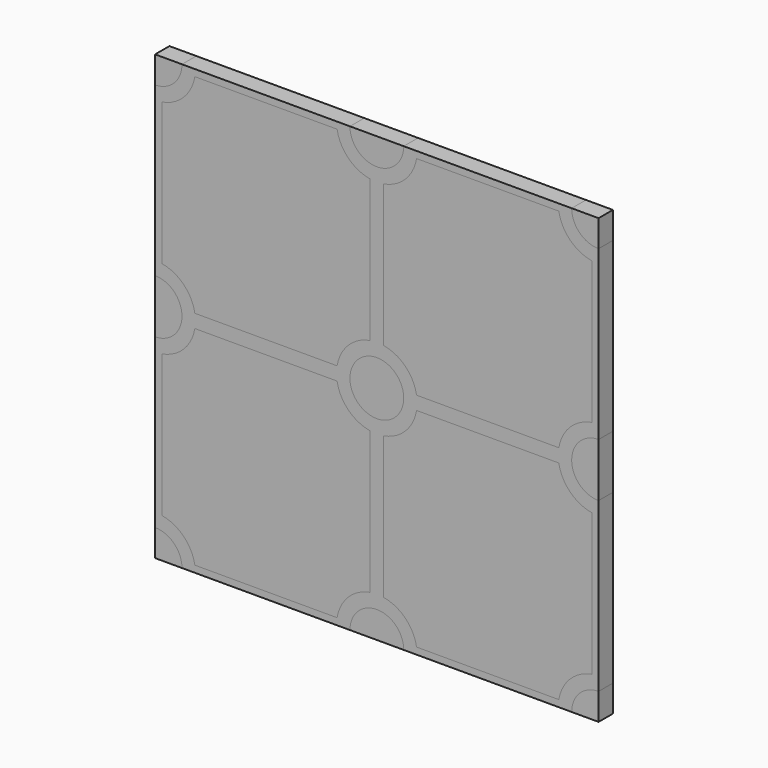
from build123d import *

# Parameters (mm, degrees)
F2_DEPTH = 6.35
F3_DEPTH = 6.35
F1_W     = 4.7625
F1_H     = 4.7625
F4_DEPTH = 6.35


with BuildPart() as f2:
    # F1 (on face) → F2 (new body)
    with BuildSketch(Plane.XZ):
        with BuildLine():
            Line((-64.4935850165, 2.38125), (-14.0876649835, 2.38125))
            ThreePointArc((-14.0876649835, 2.38125), (-10.1027881362, 10.1027881362), (-2.38125, 14.0876649835))
            Line((-2.38125, 14.0876649835), (-2.38125, 64.4935850165))
            ThreePointArc((-2.38125, 64.4935850165), (-10.1027881362, 68.4784618638), (-14.0876649835, 76.2))
            Line((-14.0876649835, 76.2), (-64.4935850165, 76.2))
            ThreePointArc((-64.4935850165, 76.2), (-68.4784618638, 68.4784618638), (-76.2, 64.4935850165))
            Line((-76.2, 64.4935850165), (-76.2, 14.0876649835))
            ThreePointArc((-76.2, 14.0876649835), (-68.4784618638, 10.1027881362), (-64.4935850165, 2.38125))
        make_face()
    extrude(amount=F2_DEPTH)


with BuildPart() as f2b:
    # F1 (on face) → F2, piece 2 (new body)
    with BuildSketch(Plane.XZ):
        with BuildLine():
            Line((14.0876649835, 2.38125), (64.4935850165, 2.38125))
            ThreePointArc((64.4935850165, 2.38125), (68.4784618638, 10.1027881362), (76.2, 14.0876649835))
            Line((76.2, 14.0876649835), (76.2, 64.4935850165))
            ThreePointArc((76.2, 64.4935850165), (68.4784618638, 68.4784618638), (64.4935850165, 76.2))
            Line((64.4935850165, 76.2), (14.0876649835, 76.2))
            ThreePointArc((14.0876649835, 76.2), (10.1027881362, 68.4784618638), (2.38125, 64.4935850165))
            Line((2.38125, 64.4935850165), (2.38125, 14.0876649835))
            ThreePointArc((2.38125, 14.0876649835), (10.1027881362, 10.1027881362), (14.0876649835, 2.38125))
        make_face()
    extrude(amount=F2_DEPTH)


with BuildPart() as f2c:
    # F1 (on face) → F2, piece 3 (new body)
    with BuildSketch(Plane.XZ):
        with BuildLine():
            Line((-64.4935850165, -76.2), (-14.0876649835, -76.2))
            ThreePointArc((-14.0876649835, -76.2), (-10.1027881362, -68.4784618638), (-2.38125, -64.4935850165))
            Line((-2.38125, -64.4935850165), (-2.38125, -14.0876649835))
            ThreePointArc((-2.38125, -14.0876649835), (-10.1027881362, -10.1027881362), (-14.0876649835, -2.38125))
            Line((-14.0876649835, -2.38125), (-64.4935850165, -2.38125))
            ThreePointArc((-64.4935850165, -2.38125), (-68.4784618638, -10.1027881362), (-76.2, -14.0876649835))
            Line((-76.2, -14.0876649835), (-76.2, -64.4935850165))
            ThreePointArc((-76.2, -64.4935850165), (-68.4784618638, -68.4784618638), (-64.4935850165, -76.2))
        make_face()
    extrude(amount=F2_DEPTH)


with BuildPart() as f2d:
    # F1 (on face) → F2, piece 4 (new body)
    with BuildSketch(Plane.XZ):
        with BuildLine():
            ThreePointArc((2.38125, -64.4935850165), (10.1027881362, -68.4784618638), (14.0876649835, -76.2))
            Line((14.0876649835, -76.2), (64.4935850165, -76.2))
            ThreePointArc((64.4935850165, -76.2), (68.4784618638, -68.4784618638), (76.2, -64.4935850165))
            Line((76.2, -64.4935850165), (76.2, -14.0876649835))
            ThreePointArc((76.2, -14.0876649835), (68.4784618638, -10.1027881362), (64.4935850165, -2.38125))
            Line((64.4935850165, -2.38125), (14.0876649835, -2.38125))
            ThreePointArc((14.0876649835, -2.38125), (10.1027881362, -10.1027881362), (2.38125, -14.0876649835))
            Line((2.38125, -14.0876649835), (2.38125, -64.4935850165))
        make_face()
    extrude(amount=F2_DEPTH)


with BuildPart() as f3:
    # F1 (on face) → F3 (new body)
    with BuildSketch(Plane.XZ):
        with BuildLine():
            Line((-76.2, 76.2), (-76.2, 69.3587084068))
            ThreePointArc((-76.2, 69.3587084068), (-71.8460579092, 71.8460579092), (-69.3587084068, 76.2))
            Line((-69.3587084068, 76.2), (-76.2, 76.2))
        make_face()
        with BuildLine():
            Line((-78.58125, 78.58125), (-78.58125, 69.05625))
            ThreePointArc((-78.58125, 69.05625), (-77.3810591141, 69.1321671431), (-76.2, 69.3587084068))
            Line((-76.2, 69.3587084068), (-76.2, 76.2))
            Line((-76.2, 76.2), (-69.3587084068, 76.2))
            ThreePointArc((-69.3587084068, 76.2), (-69.1321671431, 77.3810591141), (-69.05625, 78.58125))
            Line((-69.05625, 78.58125), (-78.58125, 78.58125))
        make_face()
    extrude(amount=F3_DEPTH)


with BuildPart() as f3b:
    # F1 (on face) → F3, piece 2 (new body)
    with BuildSketch(Plane.XZ):
        with BuildLine():
            Line((9.525, 78.58125), (-9.525, 78.58125))
            ThreePointArc((-9.525, 78.58125), (-9.4490828569, 77.3810591141), (-9.2225415932, 76.2))
            Line((-9.2225415932, 76.2), (-2.38125, 76.2))
            Line((-2.38125, 76.2), (2.38125, 76.2))
            Line((2.38125, 76.2), (9.2225415932, 76.2))
            ThreePointArc((9.2225415932, 76.2), (9.4490828569, 77.3810591141), (9.525, 78.58125))
        make_face()
        with BuildLine():
            ThreePointArc((-9.2225415932, 76.2), (-6.7351920908, 71.8460579092), (-2.38125, 69.3587084068))
            Line((-2.38125, 69.3587084068), (-2.38125, 76.2))
            Line((-2.38125, 76.2), (-9.2225415932, 76.2))
        make_face()
        with BuildLine():
            Line((-2.38125, 76.2), (-2.38125, 69.3587084068))
            ThreePointArc((-2.38125, 69.3587084068), (0, 69.05625), (2.38125, 69.3587084068))
            Line((2.38125, 69.3587084068), (2.38125, 76.2))
            Line((2.38125, 76.2), (-2.38125, 76.2))
        make_face()
        with BuildLine():
            Line((2.38125, 76.2), (2.38125, 69.3587084068))
            ThreePointArc((2.38125, 69.3587084068), (6.7351920908, 71.8460579092), (9.2225415932, 76.2))
            Line((9.2225415932, 76.2), (2.38125, 76.2))
        make_face()
    extrude(amount=F3_DEPTH)


with BuildPart() as f3c:
    # F1 (on face) → F3, piece 3 (new body)
    with BuildSketch(Plane.XZ):
        with BuildLine():
            ThreePointArc((69.3587084068, 76.2), (71.8460579092, 71.8460579092), (76.2, 69.3587084068))
            Line((76.2, 69.3587084068), (76.2, 76.2))
            Line((76.2, 76.2), (69.3587084068, 76.2))
        make_face()
        with BuildLine():
            ThreePointArc((76.2, 69.3587084068), (77.3810591141, 69.1321671431), (78.58125, 69.05625))
            Line((78.58125, 69.05625), (78.58125, 78.58125))
            Line((78.58125, 78.58125), (69.05625, 78.58125))
            ThreePointArc((69.05625, 78.58125), (69.1321671431, 77.3810591141), (69.3587084068, 76.2))
            Line((69.3587084068, 76.2), (76.2, 76.2))
            Line((76.2, 76.2), (76.2, 69.3587084068))
        make_face()
    extrude(amount=F3_DEPTH)


with BuildPart() as f3d:
    # F1 (on face) → F3, piece 4 (new body)
    with BuildSketch(Plane.XZ):
        with BuildLine():
            Line((69.3587084068, 2.38125), (76.2, 2.38125))
            Line((76.2, 2.38125), (76.2, 9.2225415932))
            ThreePointArc((76.2, 9.2225415932), (71.8460579092, 6.7351920908), (69.3587084068, 2.38125))
        make_face()
        with BuildLine():
            Line((76.2, -2.38125), (76.2, -9.2225415932))
            ThreePointArc((76.2, -9.2225415932), (77.3810591141, -9.4490828569), (78.58125, -9.525))
            Line((78.58125, -9.525), (78.58125, 9.525))
            ThreePointArc((78.58125, 9.525), (77.3810591141, 9.4490828569), (76.2, 9.2225415932))
            Line((76.2, 9.2225415932), (76.2, 2.38125))
            Line((76.2, 2.38125), (76.2, -2.38125))
        make_face()
        with BuildLine():
            Line((69.3587084068, -2.38125), (76.2, -2.38125))
            Line((76.2, -2.38125), (76.2, 2.38125))
            Line((76.2, 2.38125), (69.3587084068, 2.38125))
            ThreePointArc((69.3587084068, 2.38125), (69.05625, 0), (69.3587084068, -2.38125))
        make_face()
        with BuildLine():
            ThreePointArc((69.3587084068, -2.38125), (71.8460579092, -6.7351920908), (76.2, -9.2225415932))
            Line((76.2, -9.2225415932), (76.2, -2.38125))
            Line((76.2, -2.38125), (69.3587084068, -2.38125))
        make_face()
    extrude(amount=F3_DEPTH)


with BuildPart() as f3e:
    # F1 (on face) → F3, piece 5 (new body)
    with BuildSketch(Plane.XZ):
        with BuildLine():
            ThreePointArc((76.2, -69.3587084068), (71.8460579092, -71.8460579092), (69.3587084068, -76.2))
            Line((69.3587084068, -76.2), (76.2, -76.2))
            Line((76.2, -76.2), (76.2, -69.3587084068))
        make_face()
        with BuildLine():
            ThreePointArc((69.3587084068, -76.2), (69.1321671431, -77.3810591141), (69.05625, -78.58125))
            Line((69.05625, -78.58125), (78.58125, -78.58125))
            Line((78.58125, -78.58125), (78.58125, -69.05625))
            ThreePointArc((78.58125, -69.05625), (77.3810591141, -69.1321671431), (76.2, -69.3587084068))
            Line((76.2, -69.3587084068), (76.2, -76.2))
            Line((76.2, -76.2), (69.3587084068, -76.2))
        make_face()
    extrude(amount=F3_DEPTH)


with BuildPart() as f3f:
    # F1 (on face) → F3, piece 6 (new body)
    with BuildSketch(Plane.XZ):
        with BuildLine():
            Line((2.38125, -76.2), (9.2225415932, -76.2))
            ThreePointArc((9.2225415932, -76.2), (6.7351920908, -71.8460579092), (2.38125, -69.3587084068))
            Line((2.38125, -69.3587084068), (2.38125, -76.2))
        make_face()
        with BuildLine():
            ThreePointArc((-2.38125, -69.3587084068), (-6.7351920908, -71.8460579092), (-9.2225415932, -76.2))
            Line((-9.2225415932, -76.2), (-2.38125, -76.2))
            Line((-2.38125, -76.2), (-2.38125, -69.3587084068))
        make_face()
        with BuildLine():
            Line((-9.525, -78.58125), (9.525, -78.58125))
            ThreePointArc((9.525, -78.58125), (9.4490828569, -77.3810591141), (9.2225415932, -76.2))
            Line((9.2225415932, -76.2), (2.38125, -76.2))
            Line((2.38125, -76.2), (-2.38125, -76.2))
            Line((-2.38125, -76.2), (-9.2225415932, -76.2))
            ThreePointArc((-9.2225415932, -76.2), (-9.4490828569, -77.3810591141), (-9.525, -78.58125))
        make_face()
        with BuildLine():
            Line((-2.38125, -76.2), (2.38125, -76.2))
            Line((2.38125, -76.2), (2.38125, -69.3587084068))
            ThreePointArc((2.38125, -69.3587084068), (0, -69.05625), (-2.38125, -69.3587084068))
            Line((-2.38125, -69.3587084068), (-2.38125, -76.2))
        make_face()
    extrude(amount=F3_DEPTH)


with BuildPart() as f3g:
    # F1 (on face) → F3, piece 7 (new body)
    with BuildSketch(Plane.XZ):
        with BuildLine():
            Line((2.38125, -2.38125), (2.38125, -9.2225415932))
            ThreePointArc((2.38125, -9.2225415932), (6.7351920908, -6.7351920908), (9.2225415932, -2.38125))
            Line((9.2225415932, -2.38125), (2.38125, -2.38125))
        make_face()
        with BuildLine():
            ThreePointArc((-2.38125, -9.2225415932), (0, -9.525), (2.38125, -9.2225415932))
            Line((2.38125, -9.2225415932), (2.38125, -2.38125))
            Line((2.38125, -2.38125), (-2.38125, -2.38125))
            Line((-2.38125, -2.38125), (-2.38125, -9.2225415932))
        make_face()
        with BuildLine():
            ThreePointArc((-9.2225415932, -2.38125), (-6.7351920908, -6.7351920908), (-2.38125, -9.2225415932))
            Line((-2.38125, -9.2225415932), (-2.38125, -2.38125))
            Line((-2.38125, -2.38125), (-9.2225415932, -2.38125))
        make_face()
        with BuildLine():
            ThreePointArc((-9.2225415932, 2.38125), (-9.525, 0), (-9.2225415932, -2.38125))
            Line((-9.2225415932, -2.38125), (-2.38125, -2.38125))
            Line((-2.38125, -2.38125), (-2.38125, 2.38125))
            Line((-2.38125, 2.38125), (-9.2225415932, 2.38125))
        make_face()
        with BuildLine():
            ThreePointArc((-2.38125, 9.2225415932), (-6.7351920908, 6.7351920908), (-9.2225415932, 2.38125))
            Line((-9.2225415932, 2.38125), (-2.38125, 2.38125))
            Line((-2.38125, 2.38125), (-2.38125, 9.2225415932))
        make_face()
        with BuildLine():
            Line((-2.38125, 2.38125), (2.38125, 2.38125))
            Line((2.38125, 2.38125), (2.38125, 9.2225415932))
            ThreePointArc((2.38125, 9.2225415932), (0, 9.525), (-2.38125, 9.2225415932))
            Line((-2.38125, 9.2225415932), (-2.38125, 2.38125))
        make_face()
        with BuildLine():
            Line((2.38125, 9.2225415932), (2.38125, 2.38125))
            Line((2.38125, 2.38125), (9.2225415932, 2.38125))
            ThreePointArc((9.2225415932, 2.38125), (6.7351920908, 6.7351920908), (2.38125, 9.2225415932))
        make_face()
        with BuildLine():
            Line((2.38125, -2.38125), (9.2225415932, -2.38125))
            ThreePointArc((9.2225415932, -2.38125), (9.4490828569, -1.2001908859), (9.525, 0))
            ThreePointArc((9.525, 0), (9.4490828569, 1.2001908859), (9.2225415932, 2.38125))
            Line((9.2225415932, 2.38125), (2.38125, 2.38125))
            Line((2.38125, 2.38125), (2.38125, -2.38125))
        make_face()
        Rectangle(F1_W, F1_H)
    extrude(amount=F3_DEPTH)


with BuildPart() as f3h:
    # F1 (on face) → F3, piece 8 (new body)
    with BuildSketch(Plane.XZ):
        with BuildLine():
            Line((-76.2, -76.2), (-69.3587084068, -76.2))
            ThreePointArc((-69.3587084068, -76.2), (-71.8460579092, -71.8460579092), (-76.2, -69.3587084068))
            Line((-76.2, -69.3587084068), (-76.2, -76.2))
        make_face()
        with BuildLine():
            Line((-78.58125, -78.58125), (-69.05625, -78.58125))
            ThreePointArc((-69.05625, -78.58125), (-69.1321671431, -77.3810591141), (-69.3587084068, -76.2))
            Line((-69.3587084068, -76.2), (-76.2, -76.2))
            Line((-76.2, -76.2), (-76.2, -69.3587084068))
            ThreePointArc((-76.2, -69.3587084068), (-77.3810591141, -69.1321671431), (-78.58125, -69.05625))
            Line((-78.58125, -69.05625), (-78.58125, -78.58125))
        make_face()
    extrude(amount=F3_DEPTH)


with BuildPart() as f3i:
    # F1 (on face) → F3, piece 9 (new body)
    with BuildSketch(Plane.XZ):
        with BuildLine():
            Line((-76.2, -2.38125), (-76.2, -9.2225415932))
            ThreePointArc((-76.2, -9.2225415932), (-71.8460579092, -6.7351920908), (-69.3587084068, -2.38125))
            Line((-69.3587084068, -2.38125), (-76.2, -2.38125))
        make_face()
        with BuildLine():
            Line((-78.58125, 9.525), (-78.58125, -9.525))
            ThreePointArc((-78.58125, -9.525), (-77.3810591141, -9.4490828569), (-76.2, -9.2225415932))
            Line((-76.2, -9.2225415932), (-76.2, -2.38125))
            Line((-76.2, -2.38125), (-76.2, 2.38125))
            Line((-76.2, 2.38125), (-76.2, 9.2225415932))
            ThreePointArc((-76.2, 9.2225415932), (-77.3810591141, 9.4490828569), (-78.58125, 9.525))
        make_face()
        with BuildLine():
            Line((-76.2, -2.38125), (-69.3587084068, -2.38125))
            ThreePointArc((-69.3587084068, -2.38125), (-69.1321671431, -1.2001908859), (-69.05625, 0))
            ThreePointArc((-69.05625, 0), (-69.1321671431, 1.2001908859), (-69.3587084068, 2.38125))
            Line((-69.3587084068, 2.38125), (-76.2, 2.38125))
            Line((-76.2, 2.38125), (-76.2, -2.38125))
        make_face()
        with BuildLine():
            ThreePointArc((-69.3587084068, 2.38125), (-71.8460579092, 6.7351920908), (-76.2, 9.2225415932))
            Line((-76.2, 9.2225415932), (-76.2, 2.38125))
            Line((-76.2, 2.38125), (-69.3587084068, 2.38125))
        make_face()
    extrude(amount=F3_DEPTH)


with BuildPart() as f4:
    # F1 (on face) → F4 (new body)
    with BuildSketch(Plane.XZ):
        with BuildLine():
            ThreePointArc((-64.4935850165, 76.2), (-64.3437964057, 77.3864398063), (-64.29375, 78.58125))
            Line((-64.29375, 78.58125), (-69.05625, 78.58125))
            ThreePointArc((-69.05625, 78.58125), (-69.1321671431, 77.3810591141), (-69.3587084068, 76.2))
            Line((-69.3587084068, 76.2), (-64.4935850165, 76.2))
        make_face()
        with BuildLine():
            Line((-76.2, 69.3587084068), (-76.2, 64.4935850165))
            ThreePointArc((-76.2, 64.4935850165), (-68.4784618638, 68.4784618638), (-64.4935850165, 76.2))
            Line((-64.4935850165, 76.2), (-69.3587084068, 76.2))
            ThreePointArc((-69.3587084068, 76.2), (-71.8460579092, 71.8460579092), (-76.2, 69.3587084068))
        make_face()
        with BuildLine():
            Line((-78.58125, 69.05625), (-78.58125, 64.29375))
            ThreePointArc((-78.58125, 64.29375), (-77.3864398063, 64.3437964057), (-76.2, 64.4935850165))
            Line((-76.2, 64.4935850165), (-76.2, 69.3587084068))
            ThreePointArc((-76.2, 69.3587084068), (-77.3810591141, 69.1321671431), (-78.58125, 69.05625))
        make_face()
        with BuildLine():
            Line((-78.58125, 64.29375), (-78.58125, 14.2875))
            ThreePointArc((-78.58125, 14.2875), (-77.3864398063, 14.2374535943), (-76.2, 14.0876649835))
            Line((-76.2, 14.0876649835), (-76.2, 64.4935850165))
            ThreePointArc((-76.2, 64.4935850165), (-77.3864398063, 64.3437964057), (-78.58125, 64.29375))
        make_face()
        with BuildLine():
            ThreePointArc((-76.2, 14.0876649835), (-77.3864398063, 14.2374535943), (-78.58125, 14.2875))
            Line((-78.58125, 14.2875), (-78.58125, 9.525))
            ThreePointArc((-78.58125, 9.525), (-77.3810591141, 9.4490828569), (-76.2, 9.2225415932))
            Line((-76.2, 9.2225415932), (-76.2, 14.0876649835))
        make_face()
        with BuildLine():
            ThreePointArc((-64.4935850165, 2.38125), (-68.4784618638, 10.1027881362), (-76.2, 14.0876649835))
            Line((-76.2, 14.0876649835), (-76.2, 9.2225415932))
            ThreePointArc((-76.2, 9.2225415932), (-71.8460579092, 6.7351920908), (-69.3587084068, 2.38125))
            Line((-69.3587084068, 2.38125), (-64.4935850165, 2.38125))
        make_face()
        with BuildLine():
            Line((-69.3587084068, -2.38125), (-64.4935850165, -2.38125))
            ThreePointArc((-64.4935850165, -2.38125), (-64.3437964057, -1.1948101937), (-64.29375, 0))
            ThreePointArc((-64.29375, 0), (-64.3437964057, 1.1948101937), (-64.4935850165, 2.38125))
            Line((-64.4935850165, 2.38125), (-69.3587084068, 2.38125))
            ThreePointArc((-69.3587084068, 2.38125), (-69.1321671431, 1.2001908859), (-69.05625, 0))
            ThreePointArc((-69.05625, 0), (-69.1321671431, -1.2001908859), (-69.3587084068, -2.38125))
        make_face()
        with BuildLine():
            Line((-76.2, -9.2225415932), (-76.2, -14.0876649835))
            ThreePointArc((-76.2, -14.0876649835), (-68.4784618638, -10.1027881362), (-64.4935850165, -2.38125))
            Line((-64.4935850165, -2.38125), (-69.3587084068, -2.38125))
            ThreePointArc((-69.3587084068, -2.38125), (-71.8460579092, -6.7351920908), (-76.2, -9.2225415932))
        make_face()
        with BuildLine():
            Line((-64.4935850165, -2.38125), (-14.0876649835, -2.38125))
            ThreePointArc((-14.0876649835, -2.38125), (-14.2875, 0), (-14.0876649835, 2.38125))
            Line((-14.0876649835, 2.38125), (-64.4935850165, 2.38125))
            ThreePointArc((-64.4935850165, 2.38125), (-64.3437964057, 1.1948101937), (-64.29375, 0))
            ThreePointArc((-64.29375, 0), (-64.3437964057, -1.1948101937), (-64.4935850165, -2.38125))
        make_face()
        with BuildLine():
            ThreePointArc((-2.38125, 14.0876649835), (-10.1027881362, 10.1027881362), (-14.0876649835, 2.38125))
            Line((-14.0876649835, 2.38125), (-9.2225415932, 2.38125))
            ThreePointArc((-9.2225415932, 2.38125), (-6.7351920908, 6.7351920908), (-2.38125, 9.2225415932))
            Line((-2.38125, 9.2225415932), (-2.38125, 14.0876649835))
        make_face()
        with BuildLine():
            ThreePointArc((-14.0876649835, 2.38125), (-14.2875, 0), (-14.0876649835, -2.38125))
            Line((-14.0876649835, -2.38125), (-9.2225415932, -2.38125))
            ThreePointArc((-9.2225415932, -2.38125), (-9.525, 0), (-9.2225415932, 2.38125))
            Line((-9.2225415932, 2.38125), (-14.0876649835, 2.38125))
        make_face()
        with BuildLine():
            ThreePointArc((-14.0876649835, -2.38125), (-10.1027881362, -10.1027881362), (-2.38125, -14.0876649835))
            Line((-2.38125, -14.0876649835), (-2.38125, -9.2225415932))
            ThreePointArc((-2.38125, -9.2225415932), (-6.7351920908, -6.7351920908), (-9.2225415932, -2.38125))
            Line((-9.2225415932, -2.38125), (-14.0876649835, -2.38125))
        make_face()
        with BuildLine():
            ThreePointArc((-2.38125, -14.0876649835), (0, -14.2875), (2.38125, -14.0876649835))
            Line((2.38125, -14.0876649835), (2.38125, -9.2225415932))
            ThreePointArc((2.38125, -9.2225415932), (0, -9.525), (-2.38125, -9.2225415932))
            Line((-2.38125, -9.2225415932), (-2.38125, -14.0876649835))
        make_face()
        with BuildLine():
            Line((2.38125, -9.2225415932), (2.38125, -14.0876649835))
            ThreePointArc((2.38125, -14.0876649835), (10.1027881362, -10.1027881362), (14.0876649835, -2.38125))
            Line((14.0876649835, -2.38125), (9.2225415932, -2.38125))
            ThreePointArc((9.2225415932, -2.38125), (6.7351920908, -6.7351920908), (2.38125, -9.2225415932))
        make_face()
        with BuildLine():
            Line((9.2225415932, 2.38125), (14.0876649835, 2.38125))
            ThreePointArc((14.0876649835, 2.38125), (10.1027881362, 10.1027881362), (2.38125, 14.0876649835))
            Line((2.38125, 14.0876649835), (2.38125, 9.2225415932))
            ThreePointArc((2.38125, 9.2225415932), (6.7351920908, 6.7351920908), (9.2225415932, 2.38125))
        make_face()
        with BuildLine():
            Line((9.2225415932, -2.38125), (14.0876649835, -2.38125))
            ThreePointArc((14.0876649835, -2.38125), (14.2374535943, -1.1948101937), (14.2875, 0))
            ThreePointArc((14.2875, 0), (14.2374535943, 1.1948101937), (14.0876649835, 2.38125))
            Line((14.0876649835, 2.38125), (9.2225415932, 2.38125))
            ThreePointArc((9.2225415932, 2.38125), (9.4490828569, 1.2001908859), (9.525, 0))
            ThreePointArc((9.525, 0), (9.4490828569, -1.2001908859), (9.2225415932, -2.38125))
        make_face()
        with BuildLine():
            ThreePointArc((2.38125, 14.0876649835), (0, 14.2875), (-2.38125, 14.0876649835))
            Line((-2.38125, 14.0876649835), (-2.38125, 9.2225415932))
            ThreePointArc((-2.38125, 9.2225415932), (0, 9.525), (2.38125, 9.2225415932))
            Line((2.38125, 9.2225415932), (2.38125, 14.0876649835))
        make_face()
        with BuildLine():
            Line((-2.38125, 64.4935850165), (-2.38125, 14.0876649835))
            ThreePointArc((-2.38125, 14.0876649835), (0, 14.2875), (2.38125, 14.0876649835))
            Line((2.38125, 14.0876649835), (2.38125, 64.4935850165))
            ThreePointArc((2.38125, 64.4935850165), (0, 64.29375), (-2.38125, 64.4935850165))
        make_face()
        with BuildLine():
            ThreePointArc((-14.0876649835, 76.2), (-10.1027881362, 68.4784618638), (-2.38125, 64.4935850165))
            Line((-2.38125, 64.4935850165), (-2.38125, 69.3587084068))
            ThreePointArc((-2.38125, 69.3587084068), (-6.7351920908, 71.8460579092), (-9.2225415932, 76.2))
            Line((-9.2225415932, 76.2), (-14.0876649835, 76.2))
        make_face()
        with BuildLine():
            Line((-2.38125, 69.3587084068), (-2.38125, 64.4935850165))
            ThreePointArc((-2.38125, 64.4935850165), (0, 64.29375), (2.38125, 64.4935850165))
            Line((2.38125, 64.4935850165), (2.38125, 69.3587084068))
            ThreePointArc((2.38125, 69.3587084068), (0, 69.05625), (-2.38125, 69.3587084068))
        make_face()
        with BuildLine():
            Line((2.38125, 69.3587084068), (2.38125, 64.4935850165))
            ThreePointArc((2.38125, 64.4935850165), (10.1027881362, 68.4784618638), (14.0876649835, 76.2))
            Line((14.0876649835, 76.2), (9.2225415932, 76.2))
            ThreePointArc((9.2225415932, 76.2), (6.7351920908, 71.8460579092), (2.38125, 69.3587084068))
        make_face()
        with BuildLine():
            Line((-9.525, 78.58125), (-14.2875, 78.58125))
            ThreePointArc((-14.2875, 78.58125), (-14.2374535943, 77.3864398063), (-14.0876649835, 76.2))
            Line((-14.0876649835, 76.2), (-9.2225415932, 76.2))
            ThreePointArc((-9.2225415932, 76.2), (-9.4490828569, 77.3810591141), (-9.525, 78.58125))
        make_face()
        with BuildLine():
            Line((-14.2875, 78.58125), (-64.29375, 78.58125))
            ThreePointArc((-64.29375, 78.58125), (-64.3437964057, 77.3864398063), (-64.4935850165, 76.2))
            Line((-64.4935850165, 76.2), (-14.0876649835, 76.2))
            ThreePointArc((-14.0876649835, 76.2), (-14.2374535943, 77.3864398063), (-14.2875, 78.58125))
        make_face()
        with BuildLine():
            Line((9.2225415932, 76.2), (14.0876649835, 76.2))
            ThreePointArc((14.0876649835, 76.2), (14.2374535943, 77.3864398063), (14.2875, 78.58125))
            Line((14.2875, 78.58125), (9.525, 78.58125))
            ThreePointArc((9.525, 78.58125), (9.4490828569, 77.3810591141), (9.2225415932, 76.2))
        make_face()
        with BuildLine():
            Line((14.0876649835, 76.2), (64.4935850165, 76.2))
            ThreePointArc((64.4935850165, 76.2), (64.3437964057, 77.3864398063), (64.29375, 78.58125))
            Line((64.29375, 78.58125), (14.2875, 78.58125))
            ThreePointArc((14.2875, 78.58125), (14.2374535943, 77.3864398063), (14.0876649835, 76.2))
        make_face()
        with BuildLine():
            ThreePointArc((64.29375, 78.58125), (64.3437964057, 77.3864398063), (64.4935850165, 76.2))
            Line((64.4935850165, 76.2), (69.3587084068, 76.2))
            ThreePointArc((69.3587084068, 76.2), (69.1321671431, 77.3810591141), (69.05625, 78.58125))
            Line((69.05625, 78.58125), (64.29375, 78.58125))
        make_face()
        with BuildLine():
            ThreePointArc((64.4935850165, 76.2), (68.4784618638, 68.4784618638), (76.2, 64.4935850165))
            Line((76.2, 64.4935850165), (76.2, 69.3587084068))
            ThreePointArc((76.2, 69.3587084068), (71.8460579092, 71.8460579092), (69.3587084068, 76.2))
            Line((69.3587084068, 76.2), (64.4935850165, 76.2))
        make_face()
        with BuildLine():
            ThreePointArc((76.2, 64.4935850165), (77.3864398063, 64.3437964057), (78.58125, 64.29375))
            Line((78.58125, 64.29375), (78.58125, 69.05625))
            ThreePointArc((78.58125, 69.05625), (77.3810591141, 69.1321671431), (76.2, 69.3587084068))
            Line((76.2, 69.3587084068), (76.2, 64.4935850165))
        make_face()
        with BuildLine():
            ThreePointArc((76.2, 14.0876649835), (77.3864398063, 14.2374535943), (78.58125, 14.2875))
            Line((78.58125, 14.2875), (78.58125, 64.29375))
            ThreePointArc((78.58125, 64.29375), (77.3864398063, 64.3437964057), (76.2, 64.4935850165))
            Line((76.2, 64.4935850165), (76.2, 14.0876649835))
        make_face()
        with BuildLine():
            ThreePointArc((76.2, 9.2225415932), (77.3810591141, 9.4490828569), (78.58125, 9.525))
            Line((78.58125, 9.525), (78.58125, 14.2875))
            ThreePointArc((78.58125, 14.2875), (77.3864398063, 14.2374535943), (76.2, 14.0876649835))
            Line((76.2, 14.0876649835), (76.2, 9.2225415932))
        make_face()
        with BuildLine():
            ThreePointArc((76.2, 14.0876649835), (68.4784618638, 10.1027881362), (64.4935850165, 2.38125))
            Line((64.4935850165, 2.38125), (69.3587084068, 2.38125))
            ThreePointArc((69.3587084068, 2.38125), (71.8460579092, 6.7351920908), (76.2, 9.2225415932))
            Line((76.2, 9.2225415932), (76.2, 14.0876649835))
        make_face()
        with BuildLine():
            ThreePointArc((64.4935850165, 2.38125), (64.29375, 0), (64.4935850165, -2.38125))
            Line((64.4935850165, -2.38125), (69.3587084068, -2.38125))
            ThreePointArc((69.3587084068, -2.38125), (69.05625, 0), (69.3587084068, 2.38125))
            Line((69.3587084068, 2.38125), (64.4935850165, 2.38125))
        make_face()
        with BuildLine():
            ThreePointArc((14.2875, 0), (14.2374535943, -1.1948101937), (14.0876649835, -2.38125))
            Line((14.0876649835, -2.38125), (64.4935850165, -2.38125))
            ThreePointArc((64.4935850165, -2.38125), (64.29375, 0), (64.4935850165, 2.38125))
            Line((64.4935850165, 2.38125), (14.0876649835, 2.38125))
            ThreePointArc((14.0876649835, 2.38125), (14.2374535943, 1.1948101937), (14.2875, 0))
        make_face()
        with BuildLine():
            ThreePointArc((64.4935850165, -2.38125), (68.4784618638, -10.1027881362), (76.2, -14.0876649835))
            Line((76.2, -14.0876649835), (76.2, -9.2225415932))
            ThreePointArc((76.2, -9.2225415932), (71.8460579092, -6.7351920908), (69.3587084068, -2.38125))
            Line((69.3587084068, -2.38125), (64.4935850165, -2.38125))
        make_face()
        with BuildLine():
            Line((76.2, -9.2225415932), (76.2, -14.0876649835))
            ThreePointArc((76.2, -14.0876649835), (77.3864398063, -14.2374535943), (78.58125, -14.2875))
            Line((78.58125, -14.2875), (78.58125, -9.525))
            ThreePointArc((78.58125, -9.525), (77.3810591141, -9.4490828569), (76.2, -9.2225415932))
        make_face()
        with BuildLine():
            Line((76.2, -14.0876649835), (76.2, -64.4935850165))
            ThreePointArc((76.2, -64.4935850165), (77.3864398063, -64.3437964057), (78.58125, -64.29375))
            Line((78.58125, -64.29375), (78.58125, -14.2875))
            ThreePointArc((78.58125, -14.2875), (77.3864398063, -14.2374535943), (76.2, -14.0876649835))
        make_face()
        with BuildLine():
            ThreePointArc((78.58125, -64.29375), (77.3864398063, -64.3437964057), (76.2, -64.4935850165))
            Line((76.2, -64.4935850165), (76.2, -69.3587084068))
            ThreePointArc((76.2, -69.3587084068), (77.3810591141, -69.1321671431), (78.58125, -69.05625))
            Line((78.58125, -69.05625), (78.58125, -64.29375))
        make_face()
        with BuildLine():
            ThreePointArc((76.2, -64.4935850165), (68.4784618638, -68.4784618638), (64.4935850165, -76.2))
            Line((64.4935850165, -76.2), (69.3587084068, -76.2))
            ThreePointArc((69.3587084068, -76.2), (71.8460579092, -71.8460579092), (76.2, -69.3587084068))
            Line((76.2, -69.3587084068), (76.2, -64.4935850165))
        make_face()
        with BuildLine():
            ThreePointArc((64.4935850165, -76.2), (64.3437964057, -77.3864398063), (64.29375, -78.58125))
            Line((64.29375, -78.58125), (69.05625, -78.58125))
            ThreePointArc((69.05625, -78.58125), (69.1321671431, -77.3810591141), (69.3587084068, -76.2))
            Line((69.3587084068, -76.2), (64.4935850165, -76.2))
        make_face()
        with BuildLine():
            ThreePointArc((14.0876649835, -76.2), (14.2374535943, -77.3864398063), (14.2875, -78.58125))
            Line((14.2875, -78.58125), (64.29375, -78.58125))
            ThreePointArc((64.29375, -78.58125), (64.3437964057, -77.3864398063), (64.4935850165, -76.2))
            Line((64.4935850165, -76.2), (14.0876649835, -76.2))
        make_face()
        with BuildLine():
            Line((9.525, -78.58125), (14.2875, -78.58125))
            ThreePointArc((14.2875, -78.58125), (14.2374535943, -77.3864398063), (14.0876649835, -76.2))
            Line((14.0876649835, -76.2), (9.2225415932, -76.2))
            ThreePointArc((9.2225415932, -76.2), (9.4490828569, -77.3810591141), (9.525, -78.58125))
        make_face()
        with BuildLine():
            Line((9.2225415932, -76.2), (14.0876649835, -76.2))
            ThreePointArc((14.0876649835, -76.2), (10.1027881362, -68.4784618638), (2.38125, -64.4935850165))
            Line((2.38125, -64.4935850165), (2.38125, -69.3587084068))
            ThreePointArc((2.38125, -69.3587084068), (6.7351920908, -71.8460579092), (9.2225415932, -76.2))
        make_face()
        with BuildLine():
            Line((2.38125, -69.3587084068), (2.38125, -64.4935850165))
            ThreePointArc((2.38125, -64.4935850165), (0, -64.29375), (-2.38125, -64.4935850165))
            Line((-2.38125, -64.4935850165), (-2.38125, -69.3587084068))
            ThreePointArc((-2.38125, -69.3587084068), (0, -69.05625), (2.38125, -69.3587084068))
        make_face()
        with BuildLine():
            ThreePointArc((-2.38125, -64.4935850165), (0, -64.29375), (2.38125, -64.4935850165))
            Line((2.38125, -64.4935850165), (2.38125, -14.0876649835))
            ThreePointArc((2.38125, -14.0876649835), (0, -14.2875), (-2.38125, -14.0876649835))
            Line((-2.38125, -14.0876649835), (-2.38125, -64.4935850165))
        make_face()
        with BuildLine():
            ThreePointArc((-2.38125, -64.4935850165), (-10.1027881362, -68.4784618638), (-14.0876649835, -76.2))
            Line((-14.0876649835, -76.2), (-9.2225415932, -76.2))
            ThreePointArc((-9.2225415932, -76.2), (-6.7351920908, -71.8460579092), (-2.38125, -69.3587084068))
            Line((-2.38125, -69.3587084068), (-2.38125, -64.4935850165))
        make_face()
        with BuildLine():
            ThreePointArc((-14.0876649835, -76.2), (-14.2374535943, -77.3864398063), (-14.2875, -78.58125))
            Line((-14.2875, -78.58125), (-9.525, -78.58125))
            ThreePointArc((-9.525, -78.58125), (-9.4490828569, -77.3810591141), (-9.2225415932, -76.2))
            Line((-9.2225415932, -76.2), (-14.0876649835, -76.2))
        make_face()
        with BuildLine():
            Line((-64.29375, -78.58125), (-14.2875, -78.58125))
            ThreePointArc((-14.2875, -78.58125), (-14.2374535943, -77.3864398063), (-14.0876649835, -76.2))
            Line((-14.0876649835, -76.2), (-64.4935850165, -76.2))
            ThreePointArc((-64.4935850165, -76.2), (-64.3437964057, -77.3864398063), (-64.29375, -78.58125))
        make_face()
        with BuildLine():
            Line((-69.3587084068, -76.2), (-64.4935850165, -76.2))
            ThreePointArc((-64.4935850165, -76.2), (-68.4784618638, -68.4784618638), (-76.2, -64.4935850165))
            Line((-76.2, -64.4935850165), (-76.2, -69.3587084068))
            ThreePointArc((-76.2, -69.3587084068), (-71.8460579092, -71.8460579092), (-69.3587084068, -76.2))
        make_face()
        with BuildLine():
            ThreePointArc((-76.2, -64.4935850165), (-77.3864398063, -64.3437964057), (-78.58125, -64.29375))
            Line((-78.58125, -64.29375), (-78.58125, -69.05625))
            ThreePointArc((-78.58125, -69.05625), (-77.3810591141, -69.1321671431), (-76.2, -69.3587084068))
            Line((-76.2, -69.3587084068), (-76.2, -64.4935850165))
        make_face()
        with BuildLine():
            Line((-78.58125, -14.2875), (-78.58125, -64.29375))
            ThreePointArc((-78.58125, -64.29375), (-77.3864398063, -64.3437964057), (-76.2, -64.4935850165))
            Line((-76.2, -64.4935850165), (-76.2, -14.0876649835))
            ThreePointArc((-76.2, -14.0876649835), (-77.3864398063, -14.2374535943), (-78.58125, -14.2875))
        make_face()
        with BuildLine():
            Line((-78.58125, -9.525), (-78.58125, -14.2875))
            ThreePointArc((-78.58125, -14.2875), (-77.3864398063, -14.2374535943), (-76.2, -14.0876649835))
            Line((-76.2, -14.0876649835), (-76.2, -9.2225415932))
            ThreePointArc((-76.2, -9.2225415932), (-77.3810591141, -9.4490828569), (-78.58125, -9.525))
        make_face()
        with BuildLine():
            Line((-69.05625, -78.58125), (-64.29375, -78.58125))
            ThreePointArc((-64.29375, -78.58125), (-64.3437964057, -77.3864398063), (-64.4935850165, -76.2))
            Line((-64.4935850165, -76.2), (-69.3587084068, -76.2))
            ThreePointArc((-69.3587084068, -76.2), (-69.1321671431, -77.3810591141), (-69.05625, -78.58125))
        make_face()
    extrude(amount=F4_DEPTH)


solid = Compound([f2.part, f2b.part, f2c.part, f2d.part, f3.part, f3b.part, f3c.part, f3d.part, f3e.part, f3f.part, f3g.part, f3h.part, f3i.part, f4.part])
